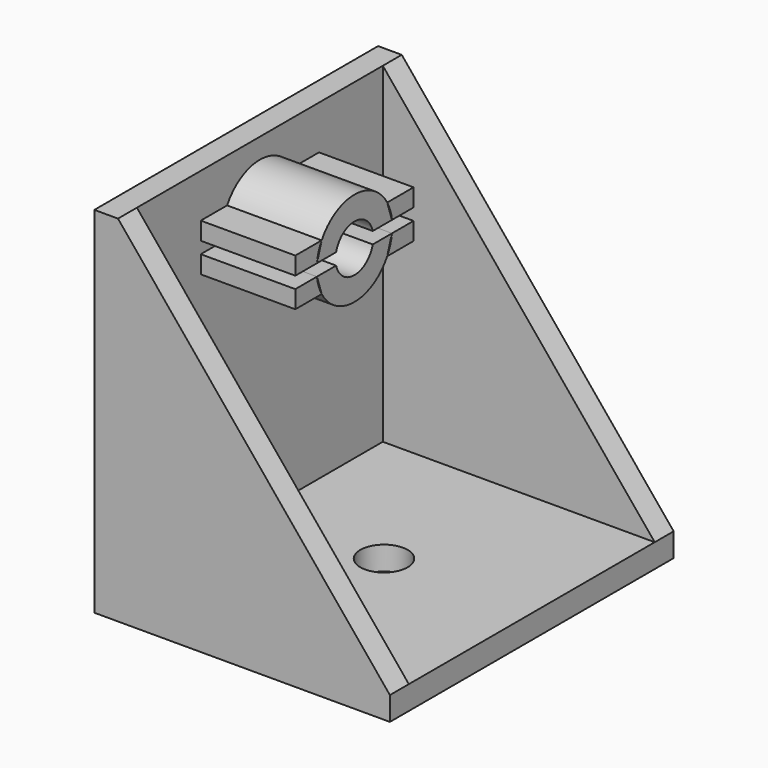
from build123d import *

# Parameters (mm, degrees)
F0_W      = 50
F0_H      = 60
F0_R      = 4
F1_DEPTH  = 4
F2_W      = 60
F2_H      = 60
F3_DEPTH  = 4
F5_DEPTH  = 4
F6_R      = 8
F6_R_2    = 4
F7_DEPTH  = 20
F8_DEPTH  = 50.001
F10_DEPTH = 46.001
F11_DEPTH = 16


# Not quite as in the source:
# - a pattern or mirror of a feature is missing from the dataset's text; its kind, count and spacing are read off the source's solid


with BuildPart() as f1:
    # F0 (on Top) → F1 (new body)
    with BuildSketch(Plane.XY):
        Rectangle(F0_W, F0_H)
        Circle(F0_R, mode=Mode.SUBTRACT)
    extrude(amount=F1_DEPTH)

    # F2 (on face) → F3 (join)
    with BuildSketch(Plane(origin=(-25, 0, 0), x_dir=(0, -1, 0), z_dir=(-1, 0, 0))):
        with Locations((0, 30)):
            Rectangle(F2_W, F2_H)
    extrude(amount=-F3_DEPTH)

    # F4 (on face) → F5 (join)
    with BuildSketch(Plane.XZ.offset(30)):
        Polygon((-21, 60), (-25, 60), (-25, 0), (25, 0), (25, 4), align=None)
    f5 = extrude(amount=-F5_DEPTH)

    # F5_copies: F5 across plane
    add(f5.mirror(Plane.ZX))

    # F6 (on face) → F7 (join)
    with BuildSketch(Plane(origin=(-25, 0, 0), x_dir=(0, -1, 0), z_dir=(-1, 0, 0))):
        with Locations((0, 48.5843531787)):
            Circle(F6_R)
        with Locations((0, 48.5843531787)):
            Circle(F6_R_2, mode=Mode.SUBTRACT)
    extrude(amount=-F7_DEPTH)

    # F6 (on face) → F8 (cut, through all)
    with BuildSketch(Plane(origin=(-25, 0, 0), x_dir=(0, -1, 0), z_dir=(-1, 0, 0))):
        with Locations((0, 48.5843531787)):
            Circle(F6_R_2)
    extrude(amount=-F8_DEPTH, mode=Mode.SUBTRACT)

    # F9 (on face) → F10 (cut, through all)
    with BuildSketch(Plane.YZ.offset(-21)):
        Polygon((12.5, 44.5843531787), (12.5, 47.5843531787), (7.9372539332, 47.5843531787), (6.9282032303, 44.5843531787), align=None)
        Polygon((7.9372539332, 47.5843531787), (12.5, 47.5843531787), (12.5, 49.5843531787), (7.9372539332, 49.5843531787), (-7.9372539332, 49.5843531787), (-12.5, 49.5843531787), (-12.5, 47.5843531787), (-7.9372539332, 47.5843531787), align=None)
        Polygon((7.9372539332, 49.5843531787), (12.5, 49.5843531787), (12.5, 52.5843531787), (6.9282032303, 52.5843531787), align=None)
        Polygon((-6.9282032303, 44.5843531787), (-7.9372539332, 47.5843531787), (-12.5, 47.5843531787), (-12.5, 44.5843531787), align=None)
        Polygon((-12.5, 49.5843531787), (-7.9372539332, 49.5843531787), (-6.9282032303, 52.5843531787), (-12.5, 52.5843531787), align=None)
    extrude(amount=F10_DEPTH, mode=Mode.SUBTRACT)


with BuildPart() as f11:
    # F9 (on face) → F11 (new body)
    with BuildSketch(Plane.YZ.offset(-21)):
        with BuildLine():
            Line((-12.5, 49.5843531787), (-7.9372539332, 49.5843531787))
            ThreePointArc((-7.9372539332, 49.5843531787), (-7.582575695, 51.1347542904), (-6.9282032303, 52.5843531787))
            Line((-6.9282032303, 52.5843531787), (-12.5, 52.5843531787))
            Line((-12.5, 52.5843531787), (-12.5, 49.5843531787))
        make_face()
    extrude(amount=F11_DEPTH)


with BuildPart() as f11b:
    # F9 (on face) → F11, piece 2 (new body)
    with BuildSketch(Plane.YZ.offset(-21)):
        with BuildLine():
            ThreePointArc((-6.9282032303, 44.5843531787), (-7.582575695, 46.0339520671), (-7.9372539332, 47.5843531787))
            Line((-7.9372539332, 47.5843531787), (-12.5, 47.5843531787))
            Line((-12.5, 47.5843531787), (-12.5, 44.5843531787))
            Line((-12.5, 44.5843531787), (-6.9282032303, 44.5843531787))
        make_face()
    extrude(amount=F11_DEPTH)


with BuildPart() as f11c:
    # F9 (on face) → F11, piece 3 (new body)
    with BuildSketch(Plane.YZ.offset(-21)):
        with BuildLine():
            Line((7.9372539332, 49.5843531787), (12.5, 49.5843531787))
            Line((12.5, 49.5843531787), (12.5, 52.5843531787))
            Line((12.5, 52.5843531787), (6.9282032303, 52.5843531787))
            ThreePointArc((6.9282032303, 52.5843531787), (7.582575695, 51.1347542904), (7.9372539332, 49.5843531787))
        make_face()
    extrude(amount=F11_DEPTH)


with BuildPart() as f11d:
    # F9 (on face) → F11, piece 4 (new body)
    with BuildSketch(Plane.YZ.offset(-21)):
        with BuildLine():
            Line((12.5, 44.5843531787), (12.5, 47.5843531787))
            Line((12.5, 47.5843531787), (7.9372539332, 47.5843531787))
            ThreePointArc((7.9372539332, 47.5843531787), (7.582575695, 46.0339520671), (6.9282032303, 44.5843531787))
            Line((6.9282032303, 44.5843531787), (12.5, 44.5843531787))
        make_face()
    extrude(amount=F11_DEPTH)


solid = Compound([f1.part, f11.part, f11b.part, f11c.part, f11d.part])
